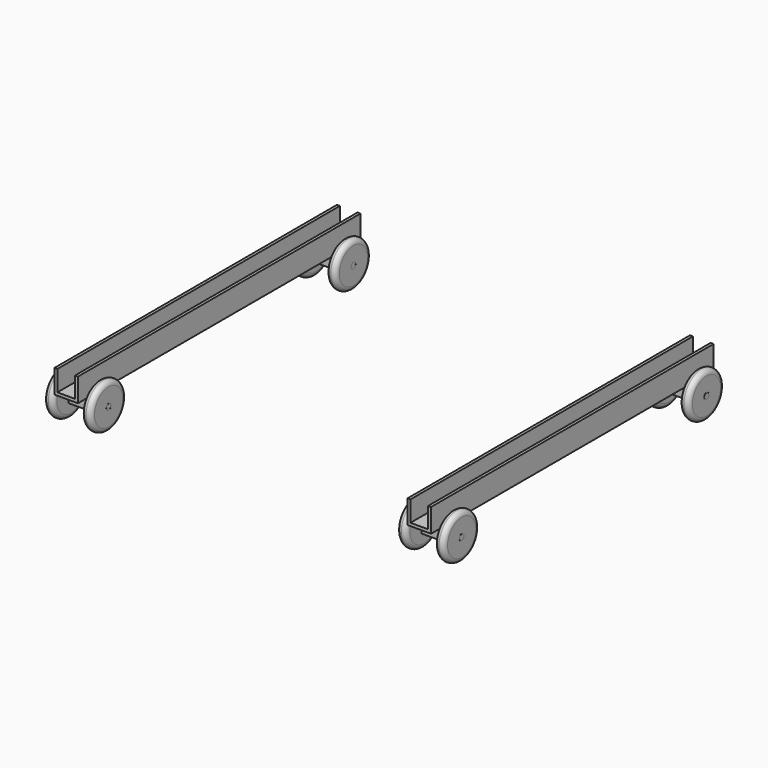
from build123d import *
from build123d import SkipClean  # not in build123d's __all__

# Parameters (mm, degrees)
F1_DEPTH      = 300
F1_DEPTH_BACK = 300
F5_DEPTH      = 40
F6_R          = 4.95
F7_DEPTH      = 40
F7_DEPTH_BACK = 40


with BuildPart() as f1:
    # F0 (on Front) → F1 (new body, two sides)
    with BuildSketch(Plane.XZ) as f1_sk:
        Polygon((-320, 0), (-280, 0), (-280, 40), (-285, 40), (-285, 5), (-315, 5), (-315, 40), (-320, 40), align=None)
    extrude(amount=F1_DEPTH)
    extrude(f1_sk.sketch, amount=-F1_DEPTH_BACK)


with BuildPart() as f1b:
    # F0 (on Front) → F1, piece 2 (new body, two sides)
    with BuildSketch(Plane.XZ) as f1_2_sk:
        Polygon((285, 5), (285, 40), (280, 40), (280, 0), (320, 0), (320, 40), (315, 40), (315, 5), align=None)
    extrude(amount=F1_DEPTH)
    extrude(f1_2_sk.sketch, amount=-F1_DEPTH_BACK)

    # F11: F5, F10, F7, F10b across plane


with BuildPart() as f5:
    # F4 (on face) → F5 (new body, through all)
    with BuildSketch(Plane(origin=(-320, 0, 0), x_dir=(0, -1, 0), z_dir=(-1, 0, 0))):
        with BuildLine():
            Line((-265, -15), (-265, 0))
            Line((-265, 0), (-270, 0))
            Line((-270, 0), (-270, -25))
            Line((-270, -25), (-250, -25))
            Line((-250, -25), (-250, 0))
            Line((-250, 0), (-255, 0))
            Line((-255, 0), (-255, -15))
            ThreePointArc((-255, -15), (-256.4644660941, -18.5355339059), (-260, -20))
            ThreePointArc((-260, -20), (-263.5355339059, -18.5355339059), (-265, -15))
        make_face()
    extrude(amount=-F5_DEPTH)


with BuildPart() as f7:
    # F6 (on plane+point) → F7 (new body, two sides)
    with BuildSketch(Plane.YZ.offset(-300)) as f7_sk:
        with Locations((260, -15.05)):
            Circle(F6_R)
    extrude(amount=F7_DEPTH)
    extrude(f7_sk.sketch, amount=-F7_DEPTH_BACK)


with BuildPart() as f10:
    # F9 (on plane+point) → F10 (revolve)
    with BuildSketch(Plane.XY.offset(-15.05)):
        with BuildLine():
            Line((-340, 265), (-332, 265))
            Line((-332, 265), (-324, 265))
            Line((-324, 265), (-324, 290))
            ThreePointArc((-324, 290), (-326.3431457505, 295.6568542495), (-332, 298))
            ThreePointArc((-332, 298), (-337.6568542495, 295.6568542495), (-340, 290))
            Line((-340, 290), (-340, 265))
        make_face()
    revolve(axis=Axis((-316, 260, -15.05), (1, 0, 0)))


with BuildPart() as f10b:
    # F9 (on plane+point) → F10, piece 2 (revolve)
    with BuildSketch(Plane.XY.offset(-15.05)):
        with BuildLine():
            Line((-268, 265), (-260, 265))
            Line((-260, 265), (-260, 290))
            ThreePointArc((-260, 290), (-262.3431457505, 295.6568542495), (-268, 298))
            ThreePointArc((-268, 298), (-273.6568542495, 295.6568542495), (-276, 290))
            Line((-276, 290), (-276, 265))
            Line((-276, 265), (-268, 265))
        make_face()
    revolve(axis=Axis((-316, 260, -15.05), (1, 0, 0)))


with BuildPart() as f1b_1:
    add(f1b.part, clean=False)
    with SkipClean():  # cleaning this boolean's faces spoils the solid; the shape is the same uncleaned
        add(f5.part.mirror(Plane.YZ), clean=False)
        add(f10.part.mirror(Plane.YZ), clean=False)
        add(f7.part.mirror(Plane.YZ), clean=False)
        add(f10b.part.mirror(Plane.YZ), clean=False)


with BuildPart() as f12_1:
    # F12: instance of F5
    add(f5.part.mirror(Plane.XZ), clean=False)


with BuildPart() as f12_2:
    # F12: instance of F1b
    add(f1b_1.part.mirror(Plane.XZ), clean=False)


with BuildPart() as f12_3:
    # F12: instance of F10b
    add(f10b.part.mirror(Plane.XZ), clean=False)


with BuildPart() as f12_4:
    # F12: instance of F7
    add(f7.part.mirror(Plane.XZ), clean=False)


with BuildPart() as f12_5:
    # F12: instance of F10
    add(f10.part.mirror(Plane.XZ), clean=False)


solid = Compound([f1.part, f5.part, f7.part, f10.part, f10b.part, f1b_1.part, f12_1.part, f12_2.part, f12_3.part, f12_4.part, f12_5.part])
